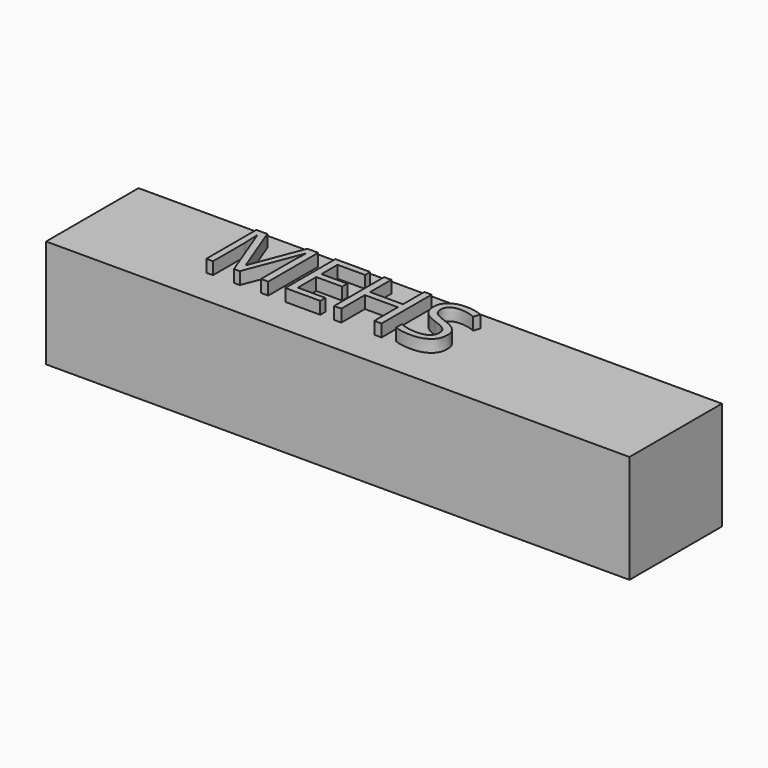
from build123d import *

# Parameters (mm, degrees)
F0_W         = 237.292945385
F0_H         = 44.0092161298
F0_R         = 12
F1_DEPTH     = 32
F2_TEXT_SIZE = 35.6270018034
F3_DEPTH     = 5
F4_W         = 237.292945385
F4_H         = 44.0092161298
F5_DEPTH     = 15


# Not quite as in the source:
# - Text() gives the source's letters only with a copy of the font that has no kerning and outlines rounded to 1/6400 em; it was checked with that copy


with BuildPart() as f1:
    # F0 (on Front) → F1 (new body)
    with BuildSketch(Plane.XZ):
        with Locations((-43.414503336, 7.7251512557)):
            Rectangle(F0_W, F0_H)
        with Locations((-125.7831007242, 8.9145898819)):
            Circle(F0_R, mode=Mode.SUBTRACT)
        with Locations((-82.3686048388, 8.9145898819)):
            Circle(F0_R, mode=Mode.SUBTRACT)
        with Locations((-38.9541052282, 8.9145898819)):
            Circle(F0_R, mode=Mode.SUBTRACT)
        with Locations((5.0551090389, 8.9145898819)):
            Circle(F0_R, mode=Mode.SUBTRACT)
        with Locations((44.9012927711, 8.9145898819)):
            Circle(F0_R, mode=Mode.SUBTRACT)
    extrude(amount=F1_DEPTH)

    # F2 (on face) → F3 (join)
    with BuildSketch(Plane.XY.offset(29.7297593206)):
        with Locations((-112.3947647704, -32)):
            Text('MEHS', F2_TEXT_SIZE, font='Open Sans', text_align=(TextAlign.LEFT, TextAlign.BOTTOM))
    extrude(amount=F3_DEPTH)

    # F4 (on face) → F5 (join)
    with BuildSketch(Plane.XZ.offset(32)):
        with Locations((-43.414503336, 7.7251512557)):
            Rectangle(F4_W, F4_H)
    extrude(amount=F5_DEPTH)


solid = f1.part
